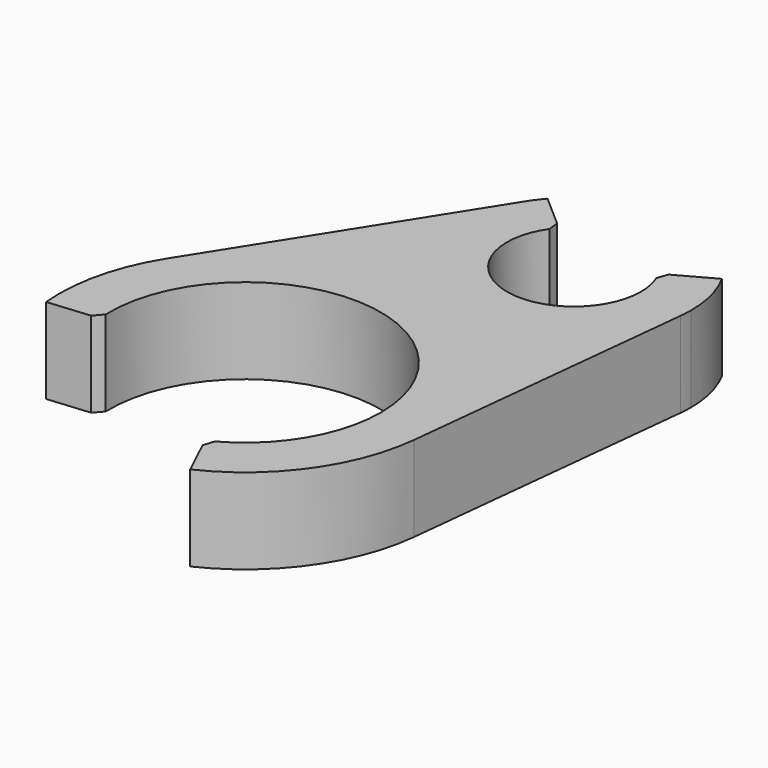
from build123d import *

# Parameters (mm, degrees)
F1_DEPTH    = 5.1
F2_T1_DEPTH = 7.5361277396
F2_T3_DEPTH = 7.6009429286


# Not quite as in the source:
# - a fillet or chamfer that OpenCascade refuses, or shapes differently, is made with other operations: its cross-section is extruded or revolved along the edge and cut away or added


with BuildPart() as f1:
    # F0 (on Top) → F1 (new body)
    with BuildSketch(Plane.XY):
        with BuildLine():
            Line((0.0307608464, 20.8328839523), (-9.3844581437, 5.9280642161))
            ThreePointArc((-9.3844581437, 5.9280642161), (-3.6624820561, 10.4783693955), (3.6482130412, 10.4833459165))
            ThreePointArc((3.6482130412, 10.4833459165), (-0.6590930389, 14.7847915444), (0.0307608464, 20.8328839523))
        make_face()
        with BuildLine():
            ThreePointArc((-8.0650120901, -0.752050521), (-0.3764319792, 8.0912482946), (8.1, 0))
            ThreePointArc((8.1, 0), (6.8438750945, -4.3325943371), (3.465092916, -7.3214159207))
            Line((3.465092916, -7.3214159207), (4.7484606627, -10.0330514468))
            ThreePointArc((4.7484606627, -10.0330514468), (9.0496936401, -6.4275224637), (11.0372396512, -1.1787030508))
            ThreePointArc((11.0372396512, -1.1787030508), (11.084298808, -0.5901863569), (11.1, 0))
            ThreePointArc((11.1, 0), (9.0472417, 6.4309733028), (3.6482130412, 10.4833459165))
            ThreePointArc((3.6482130412, 10.4833459165), (-3.6624820561, 10.4783693955), (-9.3844581437, 5.9280642161))
            ThreePointArc((-9.3844581437, 5.9280642161), (-10.7943717933, 2.586800647), (-11.052053605, -1.030587751))
            Line((-11.052053605, -1.030587751), (-8.0650120901, -0.752050521))
        make_face()
        with BuildLine():
            ThreePointArc((11.1, 0), (11.084298808, -0.5901863569), (11.0372396512, -1.1787030508))
            Line((11.0372396512, -1.1787030508), (12.9093090053, 16.351138829))
            ThreePointArc((12.9093090053, 16.351138829), (9.6953604205, 11.1814335847), (3.6482130412, 10.4833459165))
            ThreePointArc((3.6482130412, 10.4833459165), (9.0472417, 6.4309733028), (11.1, 0))
        make_face()
        with BuildLine():
            ThreePointArc((0.0307608464, 20.8328839523), (-0.6590930389, 14.7847915444), (3.6482130412, 10.4833459165))
            ThreePointArc((3.6482130412, 10.4833459165), (9.6953604205, 11.1814335847), (12.9093090053, 16.351138829))
            ThreePointArc((12.9093090053, 16.351138829), (12.938985951, 16.7222754829), (12.9488876036, 17.0944650773))
            ThreePointArc((12.9488876036, 17.0944650773), (12.7292523894, 18.8341930364), (12.0841294975, 20.4647479889))
            Line((12.0841294975, 20.4647479889), (9.4547401144, 19.0203410268))
            ThreePointArc((9.4547401144, 19.0203410268), (9.8233817669, 18.0885953396), (9.9488876036, 17.0944650773))
            ThreePointArc((9.9488876036, 17.0944650773), (4.5409128854, 13.3504555697), (2.9400840071, 19.730200443))
            Line((2.9400840071, 19.730200443), (0.6834813098, 21.7070019672))
            ThreePointArc((0.6834813098, 21.7070019672), (0.3400665642, 21.282677888), (0.0307608464, 20.8328839523))
        make_face()
    extrude(amount=F1_DEPTH)

    # F2: chamfer of 0.5 on 4 edges, made by hand

    # F2_s2 → F2_t1 (cut)
    with BuildSketch(Plane.XY.offset(-1.2180638698)):
        with BuildLine():
            Line((9.8685498702, 19.2476598469), (9.6470180572, 18.6188768158))
            ThreePointArc((9.6470180572, 18.6188768158), (9.5595268283, 18.8158843724), (9.4547401144, 19.0203410268))
            Line((9.4547401144, 19.0203410268), (9.8685498702, 19.2476598469))
        make_face()
        with BuildLine():
            Line((2.665855064, 19.3795684325), (2.5849429173, 20.0413068015))
            Line((2.5849429173, 20.0413068015), (2.9400840071, 19.730200443))
            ThreePointArc((2.9400840071, 19.730200443), (2.7937225781, 19.5531097571), (2.665855064, 19.3795684325))
        make_face()
    extrude(amount=F2_T1_DEPTH, mode=Mode.SUBTRACT)

    # F2_s4 → F2_t3 (cut)
    with BuildSketch(Plane.XY.offset(-1.2504714643)):
        with BuildLine():
            Line((3.8848953119, -7.1075726106), (3.6727644101, -7.7602062851))
            Line((3.6727644101, -7.7602062851), (3.465092916, -7.3214159207))
            ThreePointArc((3.465092916, -7.3214159207), (3.682856675, -7.2143306489), (3.8848953119, -7.1075726106))
        make_face()
        with BuildLine():
            Line((-8.5483679919, -0.7971227482), (-8.0950937203, -0.2818823506))
            ThreePointArc((-8.0950937203, -0.2818823506), (-8.0839209794, -0.5101192), (-8.0650120901, -0.752050521))
            Line((-8.0650120901, -0.752050521), (-8.5483679919, -0.7971227482))
        make_face()
    extrude(amount=F2_T3_DEPTH, mode=Mode.SUBTRACT)


solid = f1.part
